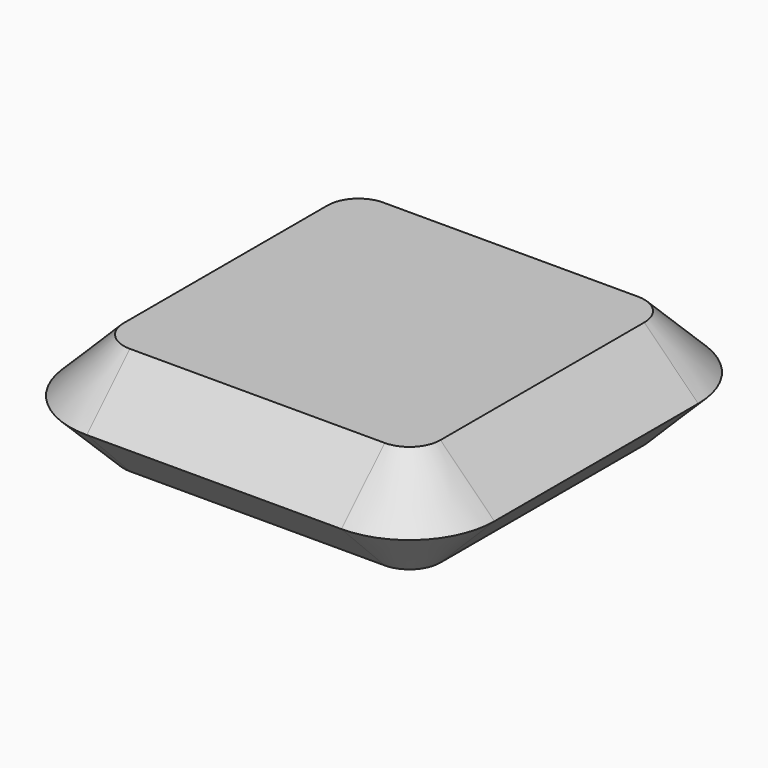
from build123d import *

# Parameters (mm, degrees)
F1_DEPTH = 25.4
F2_SIZE  = 12.69999


# Not quite as in the source:
# - a fillet or chamfer is up to 0.001 mm smaller than in the source, because OpenCascade refuses the exact size
# - a feature names something its author has since deleted; it is built from what else it names


with BuildPart() as f1:
    # F0 (on Top) → F1 (new body)
    with BuildSketch(Plane.XY):
        with BuildLine():
            Line((-30, -50), (30, -50))
            ThreePointArc((30, -50), (44.1421356237, -44.1421356237), (50, -30))
            Line((50, -30), (50, 30))
            ThreePointArc((50, 30), (44.1421356237, 44.1421356237), (30, 50))
            Line((30, 50), (-30, 50))
            ThreePointArc((-30, 50), (-44.1421356237, 44.1421356237), (-50, 30))
            Line((-50, 30), (-50, -30))
            ThreePointArc((-50, -30), (-44.1421356237, -44.1421356237), (-30, -50))
        make_face()
    extrude(amount=F1_DEPTH)

    # F2 (size 12.7 in the source; OpenCascade refuses exactly that, so slightly less here)
    f2_edges = [f1.edges().sort_by_distance(p)[0] for p in [
        (0, -50, 0),
        (44.142136, -44.142136, 0),
        (50, 0, 0),
        (44.142136, 44.142136, 0),
        (0, 50, 0),
        (-44.142136, 44.142136, 0),
        (-50, 0, 0),
        (-44.142136, -44.142136, 0),
        (0, -50, 25.4),
        (44.142136, -44.142136, 25.4),
        (50, 0, 25.4),
        (44.142136, 44.142136, 25.4),
        (0, 50, 25.4),
        (-44.142136, 44.142136, 25.4),
        (-50, 0, 25.4),
        (-44.142136, -44.142136, 25.4),
    ]]
    chamfer(f2_edges, length=F2_SIZE)


solid = f1.part
